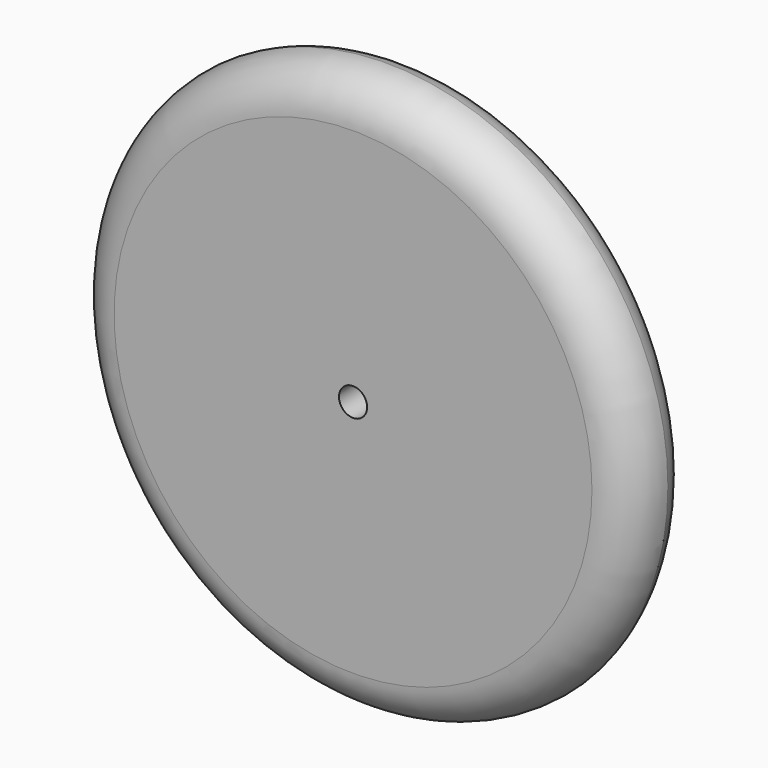
from build123d import *

# Parameters (mm, degrees)
F0_R     = 100
F1_DEPTH = 27
F2_R     = 15
F4_R     = 5
F5_DEPTH = 30


# Not quite as in the source:
# - a fillet or chamfer that OpenCascade refuses, or shapes differently, is made with other operations: its cross-section is extruded or revolved along the edge and cut away or added


with BuildPart() as f1:
    # F0 (on Front) → F1 (new body)
    with BuildSketch(Plane.XZ):
        Circle(F0_R)
    extrude(amount=F1_DEPTH)

    # F2
    f2_edges = [f1.edges().sort_by_distance(p)[0] for p in [
        (-100, -27, 0),
    ]]
    fillet(f2_edges, radius=F2_R)

    # F3: fillet of radius 15 on 1 edges, made by hand

    # F3_s1 → F3_t2 (revolve, cut)
    with BuildSketch(Plane.XY):
        with BuildLine():
            ThreePointArc((100, -12), (94.7898945238, -3.3810499614), (85.3030615433, 0))
            Line((85.3030615433, 0), (100, 0))
            Line((100, 0), (100, -12))
        make_face()
    revolve(axis=Axis((0, 0, 0), (0, -1, 0)), mode=Mode.SUBTRACT)

    # F4 (on face) → F5 (cut)
    with BuildSketch(Plane.XZ.offset(27)):
        Circle(F4_R)
    extrude(amount=-F5_DEPTH, mode=Mode.SUBTRACT)


solid = f1.part
